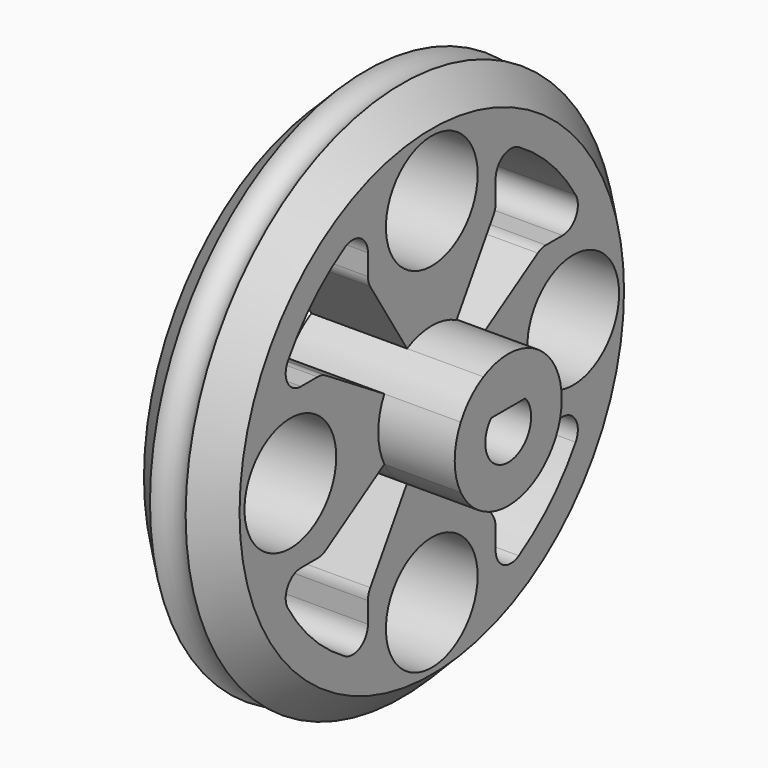
from build123d import *
from build123d import SkipClean  # not in build123d's __all__

# Parameters (mm, degrees)
F3_DEPTH = 25
F5_DEPTH = 25
F6_R     = 1
F7_R     = 3
F8_DEPTH = 25


with BuildPart() as f1:
    # F0 (on Top) → F1 (revolve)
    with BuildSketch(Plane.XY):
        with BuildLine():
            Line((-2.5, 12.5748384835), (-2.5, 0))
            Line((-2.5, 0), (6.5, 0))
            Line((6.5, 0), (6.5, 3.5))
            Line((6.5, 3.5), (2.5, 3.5))
            Line((2.5, 3.5), (2.5, 12.5748384835))
            Line((2.5, 12.5748384835), (0.9334766536, 14.1413618298))
            ThreePointArc((0.9334766536, 14.1413618298), (0, 13.5), (-0.9334766536, 14.1413618298))
            Line((-0.9334766536, 14.1413618298), (-2.5, 12.5748384835))
        make_face()
    revolve(axis=Axis((2, 0, 0), (1, 0, 0)))

    # F2 (on face) → F3 (cut)
    with BuildSketch(Plane(origin=(-2.5, 0, 0), x_dir=(0, -1, 0), z_dir=(-1, 0, 0))):
        with BuildLine():
            Line((-4.1763500472, 7.1763500472), (-4.1763500472, 10.1763500472))
            ThreePointArc((-4.1763500472, 10.1763500472), (-7.7781745931, 7.7781745931), (-10.1763500472, 4.1763500472))
            Line((-10.1763500472, 4.1763500472), (-7.1763500472, 4.1763500472))
            Line((-7.1763500472, 4.1763500472), (-3.1025807736, 1.6198742369))
            ThreePointArc((-3.1025807736, 1.6198742369), (-2.4748737342, 2.4748737342), (-1.6198742369, 3.1025807736))
            Line((-1.6198742369, 3.1025807736), (-4.1763500472, 7.1763500472))
        make_face()
        with BuildLine():
            ThreePointArc((10.1763500472, 4.1763500472), (7.7781745931, 7.7781745931), (4.1763500472, 10.1763500472))
            Line((4.1763500472, 10.1763500472), (4.1763500472, 7.1763500472))
            Line((4.1763500472, 7.1763500472), (1.6198742369, 3.1025807736))
            ThreePointArc((1.6198742369, 3.1025807736), (2.4748737342, 2.4748737342), (3.1025807736, 1.6198742369))
            Line((3.1025807736, 1.6198742369), (7.1763500472, 4.1763500472))
            Line((7.1763500472, 4.1763500472), (10.1763500472, 4.1763500472))
        make_face()
        with BuildLine():
            Line((-7.1763500472, -4.1763500472), (-10.1763500472, -4.1763500472))
            ThreePointArc((-10.1763500472, -4.1763500472), (-7.7781745931, -7.7781745931), (-4.1763500472, -10.1763500472))
            Line((-4.1763500472, -10.1763500472), (-4.1763500472, -7.1763500472))
            Line((-4.1763500472, -7.1763500472), (-1.6198742369, -3.1025807736))
            ThreePointArc((-1.6198742369, -3.1025807736), (-2.4748737342, -2.4748737342), (-3.1025807736, -1.6198742369))
            Line((-3.1025807736, -1.6198742369), (-7.1763500472, -4.1763500472))
        make_face()
        with BuildLine():
            Line((10.1763500472, -4.1763500472), (7.1763500472, -4.1763500472))
            Line((7.1763500472, -4.1763500472), (3.1025807736, -1.6198742369))
            ThreePointArc((3.1025807736, -1.6198742369), (2.4748737342, -2.4748737342), (1.6198742369, -3.1025807736))
            Line((1.6198742369, -3.1025807736), (4.1763500472, -7.1763500472))
            Line((4.1763500472, -7.1763500472), (4.1763500472, -10.1763500472))
            ThreePointArc((4.1763500472, -10.1763500472), (7.7781745931, -7.7781745931), (10.1763500472, -4.1763500472))
        make_face()
    with SkipClean():  # cleaning this boolean's faces spoils the solid; the shape is the same uncleaned
        extrude(amount=-F3_DEPTH, mode=Mode.SUBTRACT)

    # F4 (on face) → F5 (cut)
    with BuildSketch(Plane.YZ.offset(6.5)):
        with BuildLine():
            Line((1.1180339887, 1), (-1.1180339887, 1))
            ThreePointArc((-1.1180339887, 1), (0, -1.5), (1.1180339887, 1))
        make_face()
    with SkipClean():  # cleaning this boolean's faces spoils the solid; the shape is the same uncleaned
        extrude(amount=-F5_DEPTH, mode=Mode.SUBTRACT)

    # F6
    f6_edges = [f1.edges().sort_by_distance(p)[0] for p in [
        (0, -10.17635, 4.17635),
        (0, 4.17635, -10.17635),
        (0, -4.17635, -10.17635),
        (0, -10.17635, -4.17635),
        (0, 10.17635, -4.17635),
        (0, 10.17635, 4.17635),
        (0, 4.17635, 10.17635),
        (0, -4.17635, 10.17635),
        (0, -4.17635, -7.17635),
        (0, -7.17635, -4.17635),
        (0, 7.17635, -4.17635),
        (0, 4.17635, -7.17635),
        (0, -7.17635, 4.17635),
        (0, -4.17635, 7.17635),
        (0, 7.17635, 4.17635),
        (0, 4.17635, 7.17635),
    ]]
    fillet(f6_edges, radius=F6_R)

    # F7 (on face) → F8 (cut)
    with BuildSketch(Plane.YZ.offset(2.5)):
        with Locations((0, 9.25)):
            Circle(F7_R)
        with Locations((-9.25, 0)):
            Circle(F7_R)
        with Locations((9.25, 0)):
            Circle(F7_R)
        with Locations((0, -9.25)):
            Circle(F7_R)
    with SkipClean():  # cleaning this boolean's faces spoils the solid; the shape is the same uncleaned
        extrude(amount=-F8_DEPTH, mode=Mode.SUBTRACT)


solid = f1.part
